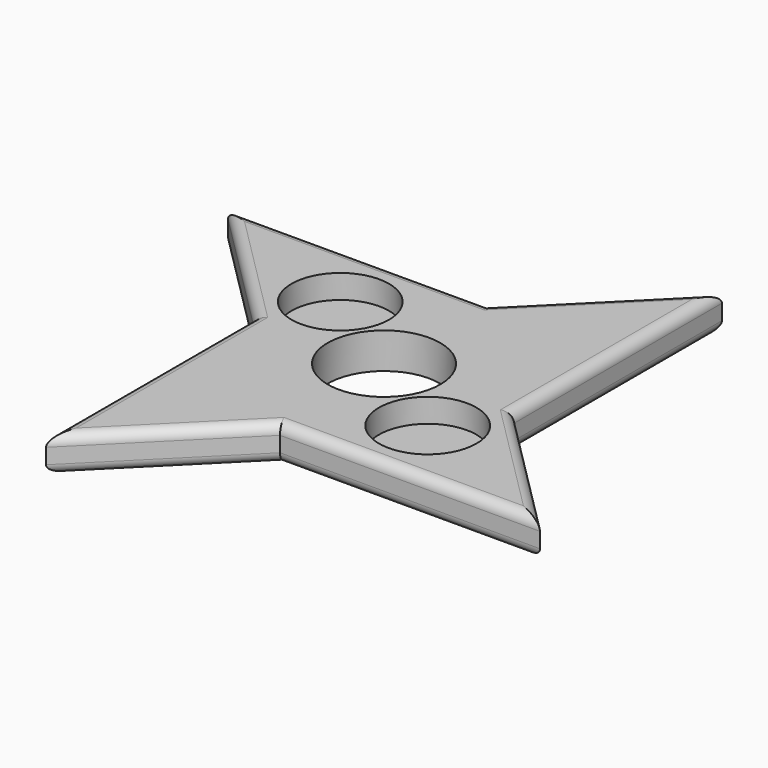
from build123d import *

# Parameters (mm, degrees)
F0_R          = 11
F1_DEPTH      = 7
F2_T4_DEPTH   = 60.8
F2_T9_DEPTH   = 45.9210244843
F2_T14_DEPTH  = 45.9210244843
F2_T19_DEPTH  = 60.8
F2_T24_DEPTH  = 45.9210244843
F2_T29_DEPTH  = 60.8
F2_T34_DEPTH  = 45.9210244843
F2_T39_DEPTH  = 60.8
F2_T44_DEPTH  = 60.8
F2_T49_DEPTH  = 45.9210244843
F2_T54_DEPTH  = 60.8
F2_T59_DEPTH  = 45.9210244843
F2_T64_DEPTH  = 60.8
F2_T69_DEPTH  = 45.9210244843
F2_T74_DEPTH  = 60.8
F2_T79_DEPTH  = 45.9210244843
F2_T85_DEPTH  = 60.8
F2_T89_DEPTH  = 45.9210244843
F2_T96_DEPTH  = 45.9210244843
F2_T100_DEPTH = 60.8
F2_T107_DEPTH = 45.9210244843
F2_T111_DEPTH = 60.8
F2_T118_DEPTH = 45.9210244843
F2_T122_DEPTH = 60.8
F2_T129_DEPTH = 60.8
F2_T133_DEPTH = 45.9210244843
F2_T140_DEPTH = 45.9210244843
F2_T144_DEPTH = 60.8
F2_T151_DEPTH = 45.9210244843
F2_T155_DEPTH = 60.8
F2_T162_DEPTH = 45.9210244843
F2_T166_DEPTH = 60.8
F3_R          = 9.525
F4_DEPTH      = 4.65
F5_R          = 9.525
F6_DEPTH      = 4.65
F7_R          = 9.525
F8_DEPTH      = 4.65
F9_R          = 9.525
F10_DEPTH     = 4.65


# Not quite as in the source:
# - a fillet or chamfer that OpenCascade refuses, or shapes differently, is made with other operations: its cross-section is extruded or revolved along the edge and cut away or added


with BuildPart() as f1:
    # F0 (on Top) → F1 (new body)
    with BuildSketch(Plane.XY):
        Polygon((-25.4, -50.8), (0, -25.4), (-25.4, -25.4), align=None)
        Polygon((25.4, 0), (25.4, 25.4), (0, 25.4), (-25.4, 25.4), (-25.4, 0), (-25.4, -25.4), (0, -25.4), (25.4, -25.4), align=None)
        Circle(F0_R, mode=Mode.SUBTRACT)
        Polygon((0, 25.4), (25.4, 25.4), (25.4, 50.8), align=None)
        Polygon((50.8, -25.4), (25.4, 0), (25.4, -25.4), align=None)
        Polygon((-25.4, 0), (-25.4, 25.4), (-50.8, 25.4), align=None)
    extrude(amount=F1_DEPTH)

    # F2: fillet of radius 2 on 20 edges, made by hand


with BuildPart() as f2_tool2:
    # F2_s3 → F2_t4 (new body)
    with BuildSketch(Plane.YZ.offset(5)):
        with BuildLine():
            ThreePointArc((25.4, 5), (24.8142135624, 6.4142135624), (23.4, 7))
            Line((23.4, 7), (25.4, 7))
            Line((25.4, 7), (25.4, 5))
        make_face()
    extrude(amount=-F2_T4_DEPTH)

    split(bisect_by=Plane(origin=(-12.7, 12.7, 0), x_dir=(0, 0, 1), z_dir=(-0.7071067812, 0.7071067812, 0)), keep=Keep.TOP)


with BuildPart() as f1_1:
    add(f1.part)

    # F2_t1: cut F2_tool2
    add(f2_tool2.part, mode=Mode.SUBTRACT)


with BuildPart() as f2_tool7:
    # F2_s8 → F2_t9 (new body)
    with BuildSketch(Plane(origin=(41.6355339059, 41.6355339059, 0), x_dir=(0, 0, 1), z_dir=(-0.7071067812, -0.7071067812, 0))):
        with BuildLine():
            ThreePointArc((5, 17.9605122421), (6.4142135624, 17.3747258045), (7, 15.9605122421))
            Line((7, 15.9605122421), (7, 17.9605122421))
            Line((7, 17.9605122421), (5, 17.9605122421))
        make_face()
    extrude(amount=F2_T9_DEPTH)

    split(bisect_by=Plane.XZ.offset(-25.4), keep=Keep.BOTTOM)


with BuildPart() as f1_2:
    add(f1_1.part)

    # F2_t6: cut F2_tool7
    add(f2_tool7.part, mode=Mode.SUBTRACT)


with BuildPart() as f2_tool12:
    # F2_s13 → F2_t14 (new body)
    with BuildSketch(Plane(origin=(-41.6355339059, 41.6355339059, 0), x_dir=(0, 0, 1), z_dir=(0.7071067812, -0.7071067812, 0))):
        with BuildLine():
            ThreePointArc((5, 17.9605122421), (6.4142135624, 17.3747258045), (7, 15.9605122421))
            Line((7, 15.9605122421), (7, 17.9605122421))
            Line((7, 17.9605122421), (5, 17.9605122421))
        make_face()
    extrude(amount=F2_T14_DEPTH)

    split(bisect_by=Plane.YZ.offset(-25.4), keep=Keep.BOTTOM)


with BuildPart() as f1_3:
    add(f1_2.part)

    # F2_t11: cut F2_tool12
    add(f2_tool12.part, mode=Mode.SUBTRACT)


with BuildPart() as f2_tool17:
    # F2_s18 → F2_t19 (new body)
    with BuildSketch(Plane.XZ.offset(-5)):
        with BuildLine():
            ThreePointArc((-25.4, 5), (-24.8142135624, 6.4142135624), (-23.4, 7))
            Line((-23.4, 7), (-25.4, 7))
            Line((-25.4, 7), (-25.4, 5))
        make_face()
    extrude(amount=F2_T19_DEPTH)

    split(bisect_by=Plane(origin=(-12.7, -12.7, 0), x_dir=(0, 0, 1), z_dir=(-0.7071067812, -0.7071067812, 0)), keep=Keep.TOP)


with BuildPart() as f1_4:
    add(f1_3.part)

    # F2_t16: cut F2_tool17
    add(f2_tool17.part, mode=Mode.SUBTRACT)


with BuildPart() as f2_tool22:
    # F2_s23 → F2_t24 (new body)
    with BuildSketch(Plane(origin=(-41.6355339059, -41.6355339059, 0), x_dir=(0, 0, 1), z_dir=(0.7071067812, 0.7071067812, 0))):
        with BuildLine():
            ThreePointArc((5, 17.9605122421), (6.4142135624, 17.3747258045), (7, 15.9605122421))
            Line((7, 15.9605122421), (7, 17.9605122421))
            Line((7, 17.9605122421), (5, 17.9605122421))
        make_face()
    extrude(amount=F2_T24_DEPTH)

    split(bisect_by=Plane.XZ.offset(25.4), keep=Keep.TOP)


with BuildPart() as f1_5:
    add(f1_4.part)

    # F2_t21: cut F2_tool22
    add(f2_tool22.part, mode=Mode.SUBTRACT)


with BuildPart() as f2_tool27:
    # F2_s28 → F2_t29 (new body)
    with BuildSketch(Plane.YZ.offset(-5)):
        with BuildLine():
            ThreePointArc((-25.4, 5), (-24.8142135624, 6.4142135624), (-23.4, 7))
            Line((-23.4, 7), (-25.4, 7))
            Line((-25.4, 7), (-25.4, 5))
        make_face()
    extrude(amount=F2_T29_DEPTH)

    split(bisect_by=Plane(origin=(12.7, -12.7, 0), x_dir=(0, 0, 1), z_dir=(0.7071067812, -0.7071067812, 0)), keep=Keep.TOP)


with BuildPart() as f1_6:
    add(f1_5.part)

    # F2_t26: cut F2_tool27
    add(f2_tool27.part, mode=Mode.SUBTRACT)


with BuildPart() as f2_tool32:
    # F2_s33 → F2_t34 (new body)
    with BuildSketch(Plane(origin=(41.6355339059, -41.6355339059, 0), x_dir=(0, 0, 1), z_dir=(-0.7071067812, 0.7071067812, 0))):
        with BuildLine():
            ThreePointArc((5, 17.9605122421), (6.4142135624, 17.3747258045), (7, 15.9605122421))
            Line((7, 15.9605122421), (7, 17.9605122421))
            Line((7, 17.9605122421), (5, 17.9605122421))
        make_face()
    extrude(amount=F2_T34_DEPTH)

    split(bisect_by=Plane.YZ.offset(25.4), keep=Keep.TOP)


with BuildPart() as f1_7:
    add(f1_6.part)

    # F2_t31: cut F2_tool32
    add(f2_tool32.part, mode=Mode.SUBTRACT)


with BuildPart() as f2_tool37:
    # F2_s38 → F2_t39 (new body)
    with BuildSketch(Plane.XZ.offset(5)):
        with BuildLine():
            ThreePointArc((25.4, 5), (24.8142135624, 6.4142135624), (23.4, 7))
            Line((23.4, 7), (25.4, 7))
            Line((25.4, 7), (25.4, 5))
        make_face()
    extrude(amount=-F2_T39_DEPTH)

    split(bisect_by=Plane(origin=(12.7, 12.7, 0), x_dir=(0, 0, 1), z_dir=(0.7071067812, 0.7071067812, 0)), keep=Keep.TOP)


with BuildPart() as f1_8:
    add(f1_7.part)

    # F2_t36: cut F2_tool37
    add(f2_tool37.part, mode=Mode.SUBTRACT)


with BuildPart() as f2_tool42:
    # F2_s43 → F2_t44 (new body)
    with BuildSketch(Plane.YZ.offset(5)):
        with BuildLine():
            ThreePointArc((25.4, 2), (24.8142135624, 0.5857864376), (23.4, 0))
            Line((23.4, 0), (25.4, 0))
            Line((25.4, 0), (25.4, 2))
        make_face()
    extrude(amount=-F2_T44_DEPTH)

    split(bisect_by=Plane(origin=(-12.7, 12.7, 0), x_dir=(0, 0, 1), z_dir=(-0.7071067812, 0.7071067812, 0)), keep=Keep.TOP)


with BuildPart() as f1_9:
    add(f1_8.part)

    # F2_t41: cut F2_tool42
    add(f2_tool42.part, mode=Mode.SUBTRACT)


with BuildPart() as f2_tool47:
    # F2_s48 → F2_t49 (new body)
    with BuildSketch(Plane(origin=(41.6355339059, 41.6355339059, 0), x_dir=(0, 0, 1), z_dir=(-0.7071067812, -0.7071067812, 0))):
        with BuildLine():
            ThreePointArc((2, 17.9605122421), (0.5857864376, 17.3747258045), (0, 15.9605122421))
            Line((0, 15.9605122421), (0, 17.9605122421))
            Line((0, 17.9605122421), (2, 17.9605122421))
        make_face()
    extrude(amount=F2_T49_DEPTH)

    split(bisect_by=Plane.XZ.offset(-25.4), keep=Keep.BOTTOM)


with BuildPart() as f1_10:
    add(f1_9.part)

    # F2_t46: cut F2_tool47
    add(f2_tool47.part, mode=Mode.SUBTRACT)


with BuildPart() as f2_tool52:
    # F2_s53 → F2_t54 (new body)
    with BuildSketch(Plane.XZ.offset(5)):
        with BuildLine():
            ThreePointArc((25.4, 2), (24.8142135624, 0.5857864376), (23.4, 0))
            Line((23.4, 0), (25.4, 0))
            Line((25.4, 0), (25.4, 2))
        make_face()
    extrude(amount=-F2_T54_DEPTH)

    split(bisect_by=Plane(origin=(12.7, 12.7, 0), x_dir=(0, 0, 1), z_dir=(0.7071067812, 0.7071067812, 0)), keep=Keep.TOP)


with BuildPart() as f1_11:
    add(f1_10.part)

    # F2_t51: cut F2_tool52
    add(f2_tool52.part, mode=Mode.SUBTRACT)


with BuildPart() as f2_tool57:
    # F2_s58 → F2_t59 (new body)
    with BuildSketch(Plane(origin=(41.6355339059, -41.6355339059, 0), x_dir=(0, 0, 1), z_dir=(-0.7071067812, 0.7071067812, 0))):
        with BuildLine():
            ThreePointArc((2, 17.9605122421), (0.5857864376, 17.3747258045), (0, 15.9605122421))
            Line((0, 15.9605122421), (0, 17.9605122421))
            Line((0, 17.9605122421), (2, 17.9605122421))
        make_face()
    extrude(amount=F2_T59_DEPTH)

    split(bisect_by=Plane.YZ.offset(25.4), keep=Keep.TOP)


with BuildPart() as f1_12:
    add(f1_11.part)

    # F2_t56: cut F2_tool57
    add(f2_tool57.part, mode=Mode.SUBTRACT)


with BuildPart() as f2_tool62:
    # F2_s63 → F2_t64 (new body)
    with BuildSketch(Plane.YZ.offset(-5)):
        with BuildLine():
            ThreePointArc((-25.4, 2), (-24.8142135624, 0.5857864376), (-23.4, 0))
            Line((-23.4, 0), (-25.4, 0))
            Line((-25.4, 0), (-25.4, 2))
        make_face()
    extrude(amount=F2_T64_DEPTH)

    split(bisect_by=Plane(origin=(12.7, -12.7, 0), x_dir=(0, 0, 1), z_dir=(0.7071067812, -0.7071067812, 0)), keep=Keep.TOP)


with BuildPart() as f1_13:
    add(f1_12.part)

    # F2_t61: cut F2_tool62
    add(f2_tool62.part, mode=Mode.SUBTRACT)


with BuildPart() as f2_tool67:
    # F2_s68 → F2_t69 (new body)
    with BuildSketch(Plane(origin=(-41.6355339059, -41.6355339059, 0), x_dir=(0, 0, 1), z_dir=(0.7071067812, 0.7071067812, 0))):
        with BuildLine():
            ThreePointArc((2, 17.9605122421), (0.5857864376, 17.3747258045), (0, 15.9605122421))
            Line((0, 15.9605122421), (0, 17.9605122421))
            Line((0, 17.9605122421), (2, 17.9605122421))
        make_face()
    extrude(amount=F2_T69_DEPTH)

    split(bisect_by=Plane.XZ.offset(25.4), keep=Keep.TOP)


with BuildPart() as f1_14:
    add(f1_13.part)

    # F2_t66: cut F2_tool67
    add(f2_tool67.part, mode=Mode.SUBTRACT)


with BuildPart() as f2_tool72:
    # F2_s73 → F2_t74 (new body)
    with BuildSketch(Plane.XZ.offset(-5)):
        with BuildLine():
            ThreePointArc((-25.4, 2), (-24.8142135624, 0.5857864376), (-23.4, 0))
            Line((-23.4, 0), (-25.4, 0))
            Line((-25.4, 0), (-25.4, 2))
        make_face()
    extrude(amount=F2_T74_DEPTH)

    split(bisect_by=Plane(origin=(-12.7, -12.7, 0), x_dir=(0, 0, 1), z_dir=(-0.7071067812, -0.7071067812, 0)), keep=Keep.TOP)


with BuildPart() as f1_15:
    add(f1_14.part)

    # F2_t71: cut F2_tool72
    add(f2_tool72.part, mode=Mode.SUBTRACT)


with BuildPart() as f2_tool77:
    # F2_s78 → F2_t79 (new body)
    with BuildSketch(Plane(origin=(-41.6355339059, 41.6355339059, 0), x_dir=(0, 0, 1), z_dir=(0.7071067812, -0.7071067812, 0))):
        with BuildLine():
            ThreePointArc((2, 17.9605122421), (0.5857864376, 17.3747258045), (0, 15.9605122421))
            Line((0, 15.9605122421), (0, 17.9605122421))
            Line((0, 17.9605122421), (2, 17.9605122421))
        make_face()
    extrude(amount=F2_T79_DEPTH)

    split(bisect_by=Plane.YZ.offset(-25.4), keep=Keep.BOTTOM)


with BuildPart() as f1_16:
    add(f1_15.part)

    # F2_t76: cut F2_tool77
    add(f2_tool77.part, mode=Mode.SUBTRACT)


with BuildPart() as f2_tool83:
    # F2_s84 → F2_t85 (new body)
    with BuildSketch(Plane.YZ.offset(5)):
        with BuildLine():
            ThreePointArc((25.4, 5), (24.8142135624, 6.4142135624), (23.4, 7))
            Line((23.4, 7), (25.4, 7))
            Line((25.4, 7), (25.4, 5))
        make_face()
    extrude(amount=-F2_T85_DEPTH)

    split(bisect_by=Plane(origin=(-12.7, 12.7, 0), x_dir=(0, 0, 1), z_dir=(0.7071067812, -0.7071067812, 0)), keep=Keep.TOP)


with BuildPart() as f2_tool87:
    # F2_s88 → F2_t89 (new body)
    with BuildSketch(Plane(origin=(41.6355339059, 41.6355339059, 0), x_dir=(0, 0, 1), z_dir=(-0.7071067812, -0.7071067812, 0))):
        with BuildLine():
            ThreePointArc((5, 17.9605122421), (6.4142135624, 17.3747258045), (7, 15.9605122421))
            Line((7, 15.9605122421), (7, 17.9605122421))
            Line((7, 17.9605122421), (5, 17.9605122421))
        make_face()
    extrude(amount=F2_T89_DEPTH)

    split(bisect_by=Plane.XZ.offset(-25.4), keep=Keep.TOP)


with BuildPart() as f2_tool83_1:
    add(f2_tool83.part)

    # F2_t91: intersect F2_tool87
    add(f2_tool87.part, mode=Mode.INTERSECT)


with BuildPart() as f1_17:
    add(f1_16.part)

    # F2_t81: cut F2_tool83
    add(f2_tool83_1.part, mode=Mode.SUBTRACT)


with BuildPart() as f2_tool94:
    # F2_s95 → F2_t96 (new body)
    with BuildSketch(Plane(origin=(-41.6355339059, 41.6355339059, 0), x_dir=(0, 0, 1), z_dir=(0.7071067812, -0.7071067812, 0))):
        with BuildLine():
            ThreePointArc((5, 17.9605122421), (6.4142135624, 17.3747258045), (7, 15.9605122421))
            Line((7, 15.9605122421), (7, 17.9605122421))
            Line((7, 17.9605122421), (5, 17.9605122421))
        make_face()
    extrude(amount=F2_T96_DEPTH)

    split(bisect_by=Plane.YZ.offset(-25.4), keep=Keep.TOP)


with BuildPart() as f2_tool98:
    # F2_s99 → F2_t100 (new body)
    with BuildSketch(Plane.XZ.offset(-5)):
        with BuildLine():
            ThreePointArc((-25.4, 5), (-24.8142135624, 6.4142135624), (-23.4, 7))
            Line((-23.4, 7), (-25.4, 7))
            Line((-25.4, 7), (-25.4, 5))
        make_face()
    extrude(amount=F2_T100_DEPTH)

    split(bisect_by=Plane(origin=(-12.7, -12.7, 0), x_dir=(0, 0, 1), z_dir=(0.7071067812, 0.7071067812, 0)), keep=Keep.TOP)


with BuildPart() as f2_tool94_1:
    add(f2_tool94.part)

    # F2_t102: intersect F2_tool98
    add(f2_tool98.part, mode=Mode.INTERSECT)


with BuildPart() as f1_18:
    add(f1_17.part)

    # F2_t92: cut F2_tool94
    add(f2_tool94_1.part, mode=Mode.SUBTRACT)


with BuildPart() as f2_tool105:
    # F2_s106 → F2_t107 (new body)
    with BuildSketch(Plane(origin=(-41.6355339059, -41.6355339059, 0), x_dir=(0, 0, 1), z_dir=(0.7071067812, 0.7071067812, 0))):
        with BuildLine():
            ThreePointArc((5, 17.9605122421), (6.4142135624, 17.3747258045), (7, 15.9605122421))
            Line((7, 15.9605122421), (7, 17.9605122421))
            Line((7, 17.9605122421), (5, 17.9605122421))
        make_face()
    extrude(amount=F2_T107_DEPTH)

    split(bisect_by=Plane.XZ.offset(25.4), keep=Keep.BOTTOM)


with BuildPart() as f2_tool109:
    # F2_s110 → F2_t111 (new body)
    with BuildSketch(Plane.YZ.offset(-5)):
        with BuildLine():
            ThreePointArc((-25.4, 5), (-24.8142135624, 6.4142135624), (-23.4, 7))
            Line((-23.4, 7), (-25.4, 7))
            Line((-25.4, 7), (-25.4, 5))
        make_face()
    extrude(amount=F2_T111_DEPTH)

    split(bisect_by=Plane(origin=(12.7, -12.7, 0), x_dir=(0, 0, 1), z_dir=(-0.7071067812, 0.7071067812, 0)), keep=Keep.TOP)


with BuildPart() as f2_tool105_1:
    add(f2_tool105.part)

    # F2_t113: intersect F2_tool109
    add(f2_tool109.part, mode=Mode.INTERSECT)


with BuildPart() as f1_19:
    add(f1_18.part)

    # F2_t103: cut F2_tool105
    add(f2_tool105_1.part, mode=Mode.SUBTRACT)


with BuildPart() as f2_tool116:
    # F2_s117 → F2_t118 (new body)
    with BuildSketch(Plane(origin=(41.6355339059, -41.6355339059, 0), x_dir=(0, 0, 1), z_dir=(-0.7071067812, 0.7071067812, 0))):
        with BuildLine():
            ThreePointArc((5, 17.9605122421), (6.4142135624, 17.3747258045), (7, 15.9605122421))
            Line((7, 15.9605122421), (7, 17.9605122421))
            Line((7, 17.9605122421), (5, 17.9605122421))
        make_face()
    extrude(amount=F2_T118_DEPTH)

    split(bisect_by=Plane.YZ.offset(25.4), keep=Keep.BOTTOM)


with BuildPart() as f2_tool120:
    # F2_s121 → F2_t122 (new body)
    with BuildSketch(Plane.XZ.offset(5)):
        with BuildLine():
            ThreePointArc((25.4, 5), (24.8142135624, 6.4142135624), (23.4, 7))
            Line((23.4, 7), (25.4, 7))
            Line((25.4, 7), (25.4, 5))
        make_face()
    extrude(amount=-F2_T122_DEPTH)

    split(bisect_by=Plane(origin=(12.7, 12.7, 0), x_dir=(0, 0, 1), z_dir=(-0.7071067812, -0.7071067812, 0)), keep=Keep.TOP)


with BuildPart() as f2_tool116_1:
    add(f2_tool116.part)

    # F2_t124: intersect F2_tool120
    add(f2_tool120.part, mode=Mode.INTERSECT)


with BuildPart() as f1_20:
    add(f1_19.part)

    # F2_t114: cut F2_tool116
    add(f2_tool116_1.part, mode=Mode.SUBTRACT)


with BuildPart() as f2_tool127:
    # F2_s128 → F2_t129 (new body)
    with BuildSketch(Plane.YZ.offset(5)):
        with BuildLine():
            ThreePointArc((25.4, 2), (24.8142135624, 0.5857864376), (23.4, 0))
            Line((23.4, 0), (25.4, 0))
            Line((25.4, 0), (25.4, 2))
        make_face()
    extrude(amount=-F2_T129_DEPTH)

    split(bisect_by=Plane(origin=(-12.7, 12.7, 0), x_dir=(0, 0, 1), z_dir=(0.7071067812, -0.7071067812, 0)), keep=Keep.TOP)


with BuildPart() as f2_tool131:
    # F2_s132 → F2_t133 (new body)
    with BuildSketch(Plane(origin=(41.6355339059, 41.6355339059, 0), x_dir=(0, 0, 1), z_dir=(-0.7071067812, -0.7071067812, 0))):
        with BuildLine():
            ThreePointArc((2, 17.9605122421), (0.5857864376, 17.3747258045), (0, 15.9605122421))
            Line((0, 15.9605122421), (0, 17.9605122421))
            Line((0, 17.9605122421), (2, 17.9605122421))
        make_face()
    extrude(amount=F2_T133_DEPTH)

    split(bisect_by=Plane.XZ.offset(-25.4), keep=Keep.TOP)


with BuildPart() as f2_tool127_1:
    add(f2_tool127.part)

    # F2_t135: intersect F2_tool131
    add(f2_tool131.part, mode=Mode.INTERSECT)


with BuildPart() as f1_21:
    add(f1_20.part)

    # F2_t125: cut F2_tool127
    add(f2_tool127_1.part, mode=Mode.SUBTRACT)


with BuildPart() as f2_tool138:
    # F2_s139 → F2_t140 (new body)
    with BuildSketch(Plane(origin=(41.6355339059, -41.6355339059, 0), x_dir=(0, 0, 1), z_dir=(-0.7071067812, 0.7071067812, 0))):
        with BuildLine():
            ThreePointArc((2, 17.9605122421), (0.5857864376, 17.3747258045), (0, 15.9605122421))
            Line((0, 15.9605122421), (0, 17.9605122421))
            Line((0, 17.9605122421), (2, 17.9605122421))
        make_face()
    extrude(amount=F2_T140_DEPTH)

    split(bisect_by=Plane.YZ.offset(25.4), keep=Keep.BOTTOM)


with BuildPart() as f2_tool142:
    # F2_s143 → F2_t144 (new body)
    with BuildSketch(Plane.XZ.offset(5)):
        with BuildLine():
            ThreePointArc((25.4, 2), (24.8142135624, 0.5857864376), (23.4, 0))
            Line((23.4, 0), (25.4, 0))
            Line((25.4, 0), (25.4, 2))
        make_face()
    extrude(amount=-F2_T144_DEPTH)

    split(bisect_by=Plane(origin=(12.7, 12.7, 0), x_dir=(0, 0, 1), z_dir=(-0.7071067812, -0.7071067812, 0)), keep=Keep.TOP)


with BuildPart() as f2_tool138_1:
    add(f2_tool138.part)

    # F2_t146: intersect F2_tool142
    add(f2_tool142.part, mode=Mode.INTERSECT)


with BuildPart() as f1_22:
    add(f1_21.part)

    # F2_t136: cut F2_tool138
    add(f2_tool138_1.part, mode=Mode.SUBTRACT)


with BuildPart() as f2_tool149:
    # F2_s150 → F2_t151 (new body)
    with BuildSketch(Plane(origin=(-41.6355339059, -41.6355339059, 0), x_dir=(0, 0, 1), z_dir=(0.7071067812, 0.7071067812, 0))):
        with BuildLine():
            ThreePointArc((2, 17.9605122421), (0.5857864376, 17.3747258045), (0, 15.9605122421))
            Line((0, 15.9605122421), (0, 17.9605122421))
            Line((0, 17.9605122421), (2, 17.9605122421))
        make_face()
    extrude(amount=F2_T151_DEPTH)

    split(bisect_by=Plane.XZ.offset(25.4), keep=Keep.BOTTOM)


with BuildPart() as f2_tool153:
    # F2_s154 → F2_t155 (new body)
    with BuildSketch(Plane.YZ.offset(-5)):
        with BuildLine():
            ThreePointArc((-25.4, 2), (-24.8142135624, 0.5857864376), (-23.4, 0))
            Line((-23.4, 0), (-25.4, 0))
            Line((-25.4, 0), (-25.4, 2))
        make_face()
    extrude(amount=F2_T155_DEPTH)

    split(bisect_by=Plane(origin=(12.7, -12.7, 0), x_dir=(0, 0, 1), z_dir=(-0.7071067812, 0.7071067812, 0)), keep=Keep.TOP)


with BuildPart() as f2_tool149_1:
    add(f2_tool149.part)

    # F2_t157: intersect F2_tool153
    add(f2_tool153.part, mode=Mode.INTERSECT)


with BuildPart() as f1_23:
    add(f1_22.part)

    # F2_t147: cut F2_tool149
    add(f2_tool149_1.part, mode=Mode.SUBTRACT)


with BuildPart() as f2_tool160:
    # F2_s161 → F2_t162 (new body)
    with BuildSketch(Plane(origin=(-41.6355339059, 41.6355339059, 0), x_dir=(0, 0, 1), z_dir=(0.7071067812, -0.7071067812, 0))):
        with BuildLine():
            ThreePointArc((2, 17.9605122421), (0.5857864376, 17.3747258045), (0, 15.9605122421))
            Line((0, 15.9605122421), (0, 17.9605122421))
            Line((0, 17.9605122421), (2, 17.9605122421))
        make_face()
    extrude(amount=F2_T162_DEPTH)

    split(bisect_by=Plane.YZ.offset(-25.4), keep=Keep.TOP)


with BuildPart() as f2_tool164:
    # F2_s165 → F2_t166 (new body)
    with BuildSketch(Plane.XZ.offset(-5)):
        with BuildLine():
            ThreePointArc((-25.4, 2), (-24.8142135624, 0.5857864376), (-23.4, 0))
            Line((-23.4, 0), (-25.4, 0))
            Line((-25.4, 0), (-25.4, 2))
        make_face()
    extrude(amount=F2_T166_DEPTH)

    split(bisect_by=Plane(origin=(-12.7, -12.7, 0), x_dir=(0, 0, 1), z_dir=(0.7071067812, 0.7071067812, 0)), keep=Keep.TOP)


with BuildPart() as f2_tool160_1:
    add(f2_tool160.part)

    # F2_t168: intersect F2_tool164
    add(f2_tool164.part, mode=Mode.INTERSECT)


with BuildPart() as f1_24:
    add(f1_23.part)

    # F2_t158: cut F2_tool160
    add(f2_tool160_1.part, mode=Mode.SUBTRACT)

    # F3 (on face) → F4 (cut)
    with BuildSketch(Plane.XY.offset(7)):
        with Locations((17.9949663132, -11.8113001988)):
            Circle(F3_R)
    extrude(amount=-F4_DEPTH, mode=Mode.SUBTRACT)

    # F5 (on face) → F6 (cut)
    with BuildSketch(Plane.XY.offset(7)):
        with Locations((-17.9949663132, 11.8113001988)):
            Circle(F5_R)
    extrude(amount=-F6_DEPTH, mode=Mode.SUBTRACT)

    # F7 (on face) → F8 (cut)
    with BuildSketch(Plane(origin=(0, 0, 0), x_dir=(1, 0, 0), z_dir=(0, 0, -1))):
        with Locations((-11.8113001988, 17.9949663132)):
            Circle(F7_R)
    extrude(amount=-F8_DEPTH, mode=Mode.SUBTRACT)

    # F9 (on face) → F10 (cut)
    with BuildSketch(Plane(origin=(0, 0, 0), x_dir=(1, 0, 0), z_dir=(0, 0, -1))):
        with Locations((11.8113001988, -17.9949663132)):
            Circle(F9_R)
    extrude(amount=-F10_DEPTH, mode=Mode.SUBTRACT)


solid = f1_24.part
